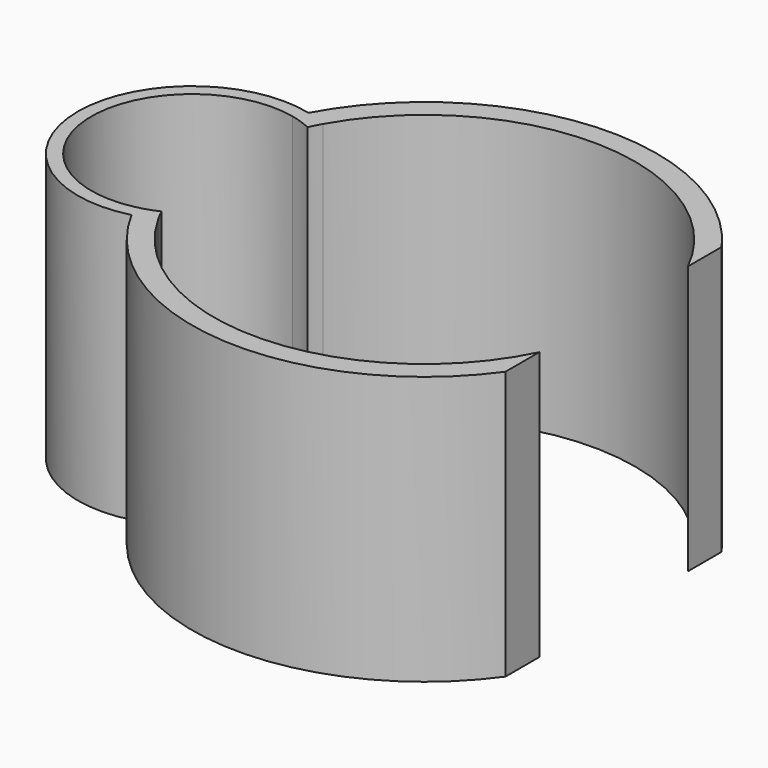
from build123d import *

# Parameters (mm, degrees)
F1_DEPTH = 10
F6_DEPTH = 10


# Not quite as in the source:
# - a feature names something its author has since deleted; it is built from what else it names


with BuildPart() as f1:
    # F0 (on Top) → F1 (new body)
    with BuildSketch(Plane.XY):
        with BuildLine():
            ThreePointArc((-7.0759814838, 3.3989683789), (-6.9640481468, 3.6227797903), (-6.8450379627, 3.8429097425))
            ThreePointArc((-6.8450379627, 3.8429097425), (-7.2244510067, 4.0001671481), (-7.6172716975, 4.1200673333))
            ThreePointArc((-7.6172716975, 4.1200673333), (-7.7361486016, 3.8922728268), (-7.8482152186, 3.6610518743))
            ThreePointArc((-7.8482152186, 3.6610518743), (-7.4549529061, 3.5510643093), (-7.0759814838, 3.3989683789))
        make_face()
        with BuildLine():
            ThreePointArc((-7.6172716975, -4.1200673333), (-7.2244510067, -4.0001671481), (-6.8450379627, -3.8429097425))
            ThreePointArc((-6.8450379627, -3.8429097425), (-6.9640481468, -3.6227797903), (-7.0759814838, -3.3989683789))
            ThreePointArc((-7.0759814838, -3.3989683789), (-7.4549529061, -3.5510643093), (-7.8482152186, -3.6610518743))
            ThreePointArc((-7.8482152186, -3.6610518743), (-7.7361486016, -3.8922728268), (-7.6172716975, -4.1200673333))
        make_face()
        with BuildLine():
            ThreePointArc((-7.8482152186, 3.6610518743), (-7.7361486016, 3.8922728268), (-7.6172716975, 4.1200673333))
            ThreePointArc((-7.6172716975, 4.1200673333), (-12.9101260351, 0), (-7.6172716975, -4.1200673333))
            ThreePointArc((-7.6172716975, -4.1200673333), (-7.7361486016, -3.8922728268), (-7.8482152186, -3.6610518743))
            ThreePointArc((-7.8482152186, -3.6610518743), (-12.4101260351, 0), (-7.8482152186, 3.6610518743))
        make_face()
    extrude(amount=F1_DEPTH)


with BuildPart() as f2_1:
    # F2: copy of F1
    add(f1.part.moved(Location((-14.3, 0, 0))))


with BuildPart() as f3_1:
    # F3: copy of F2_1
    add(f2_1.part.moved(Location((-13, 0, 0))))


with BuildPart() as f1_1:
    add(f1.part)

    # F0 (on Top) → F6 (join)
    with BuildSketch(Plane.XY):
        with BuildLine():
            ThreePointArc((-6.8450379627, 3.8429097425), (0.2165563909, 7.8470123824), (7.0465658628, 3.4595389203))
            Line((7.0465658628, 3.4595389203), (7.0465658628, 5.0342519291))
            ThreePointArc((7.0465658628, 5.0342519291), (-0.5388503097, 8.6433456073), (-7.6172716975, 4.1200673333))
            ThreePointArc((-7.6172716975, 4.1200673333), (-7.2244510067, 4.0001671481), (-6.8450379627, 3.8429097425))
        make_face()
        with BuildLine():
            Line((7.0465658628, -5.0342519291), (7.0465658628, -3.4595389203))
            ThreePointArc((7.0465658628, -3.4595389203), (0.2165563909, -7.8470123824), (-6.8450379627, -3.8429097425))
            ThreePointArc((-6.8450379627, -3.8429097425), (-7.2244510067, -4.0001671481), (-7.6172716975, -4.1200673333))
            ThreePointArc((-7.6172716975, -4.1200673333), (-0.5388503097, -8.6433456073), (7.0465658628, -5.0342519291))
        make_face()
        with BuildLine():
            ThreePointArc((-7.0759814838, 3.3989683789), (-6.9640481468, 3.6227797903), (-6.8450379627, 3.8429097425))
            ThreePointArc((-6.8450379627, 3.8429097425), (-7.2244510067, 4.0001671481), (-7.6172716975, 4.1200673333))
            ThreePointArc((-7.6172716975, 4.1200673333), (-7.7361486016, 3.8922728268), (-7.8482152186, 3.6610518743))
            ThreePointArc((-7.8482152186, 3.6610518743), (-7.4549529061, 3.5510643093), (-7.0759814838, 3.3989683789))
        make_face()
        with BuildLine():
            ThreePointArc((-7.6172716975, -4.1200673333), (-7.2244510067, -4.0001671481), (-6.8450379627, -3.8429097425))
            ThreePointArc((-6.8450379627, -3.8429097425), (-6.9640481468, -3.6227797903), (-7.0759814838, -3.3989683789))
            ThreePointArc((-7.0759814838, -3.3989683789), (-7.4549529061, -3.5510643093), (-7.8482152186, -3.6610518743))
            ThreePointArc((-7.8482152186, -3.6610518743), (-7.7361486016, -3.8922728268), (-7.6172716975, -4.1200673333))
        make_face()
    extrude(amount=F6_DEPTH)


with BuildPart() as f7_1:
    # F7: copy of F1
    add(f1_1.part.moved(Location((-22.5, 0, 0))))


with BuildPart() as f8_1:
    # F8: copy of F1
    add(f1_1.part.moved(Location((0, 18.6, 0))))


with BuildPart() as f9_1:
    # F9: copy of F7_1
    add(f7_1.part.moved(Location((0, 20.1, 0))))


with BuildPart() as f10_1:
    # F10: copy of F7_1
    add(f7_1.part.moved(Location((0, -19.2, 0))))


with BuildPart() as f11_1:
    # F11: copy of F1
    add(f1_1.part.moved(Location((0, -19.5, 0))))


with BuildPart() as f12_1:
    # F12: copy of F1
    add(f1_1.part.moved(Location((25.2, 0, 0))))


solid = f1_1.part
